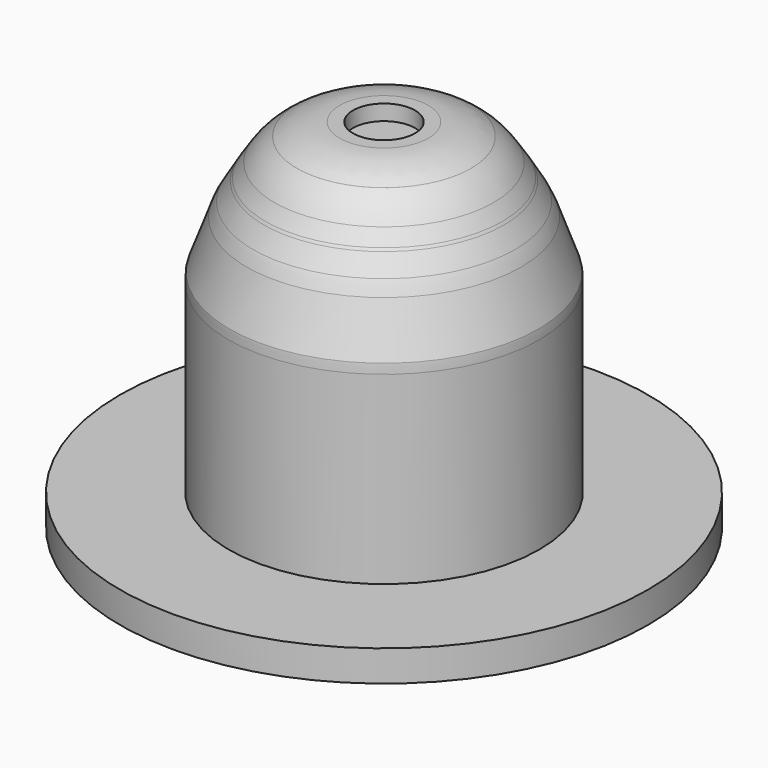
from build123d import *

# Parameters (mm, degrees)
F0_R     = 43.18
F0_R_2   = 25.4
F1_DEPTH = 5.08
F2_DEPTH = 36.83
F6_R     = 5.08
F7_DEPTH = 2.54


# Not quite as in the source:
# - a fillet or chamfer that OpenCascade refuses, or shapes differently, is made with other operations: its cross-section is extruded or revolved along the edge and cut away or added


with BuildPart() as f1:
    # F0 (on Top) → F1 (new body)
    with BuildSketch(Plane.XY):
        Circle(F0_R)
        Circle(F0_R_2, mode=Mode.SUBTRACT)
    extrude(amount=F1_DEPTH)

    # F0 (on Top) → F2 (join)
    with BuildSketch(Plane.XY):
        Circle(F0_R_2)
    extrude(amount=F2_DEPTH)

    # F3 (on Front) → F4 (revolve)
    with BuildSketch(Plane.XZ):
        Polygon((0, 58.42), (0, 36.8297025561), (25.3384895623, 36.7359854281), (22.0302641392, 45.9328517318), (19.5160117, 50.1673817635), (16.4724439383, 54.8650622368), (11.0508995131, 58.42), align=None)
    revolve(axis=Axis((0, 0, 47.6248512781), (0, 0, 1)))

    # F5: fillet of radius 12.7 on 5 edges, made by hand

    # F5_s1 → F5_t2 (revolve, cut)
    with BuildSketch(Plane.XZ):
        with BuildLine():
            ThreePointArc((25.4, 35.2768549118), (25.3761454392, 36.0548888463), (25.3046713696, 36.83))
            Line((25.3046713696, 36.83), (25.4, 36.83))
            Line((25.4, 36.83), (25.4, 35.2768549118))
        make_face()
    revolve(axis=Axis((0, 0, 36.83), (0, 0, 1)), mode=Mode.SUBTRACT)

    # F5_s3 → F5_t4 (revolve, cut)
    with BuildSketch(Plane.XZ):
        with BuildLine():
            ThreePointArc((19.6427134925, 49.9539892906), (19.513951513, 50.166103437), (19.3810699459, 50.3756614184))
            Line((19.3810699459, 50.3756614184), (19.5160117, 50.1673817635))
            Line((19.5160117, 50.1673817635), (19.6427134925, 49.9539892906))
        make_face()
    revolve(axis=Axis((0, 0, 50.1673817635), (0, 0, 1)), mode=Mode.SUBTRACT)

    # F5_s5 → F5_t6 (revolve, cut)
    with BuildSketch(Plane.XZ):
        with BuildLine():
            ThreePointArc((22.4409800917, 44.79106143), (21.9779508662, 45.9081881165), (21.4107694035, 46.9762111901))
            Line((21.4107694035, 46.9762111901), (22.0302641392, 45.9328517318))
            Line((22.0302641392, 45.9328517318), (22.4409800917, 44.79106143))
        make_face()
    revolve(axis=Axis((0, 0, 45.9328517318), (0, 0, 1)), mode=Mode.SUBTRACT)

    # F5_s7 → F5_t8 (revolve, cut)
    with BuildSketch(Plane.XZ):
        with BuildLine():
            ThreePointArc((17.9281816755, 52.6181627827), (16.274530798, 54.6682321185), (14.2335662066, 56.3331072017))
            Line((14.2335662066, 56.3331072017), (16.4724439383, 54.8650622368))
            Line((16.4724439383, 54.8650622368), (17.9281816755, 52.6181627827))
        make_face()
    revolve(axis=Axis((0, 0, 54.8650622368), (0, 0, 1)), mode=Mode.SUBTRACT)

    # F5_s9 → F5_t10 (revolve, cut)
    with BuildSketch(Plane.XZ):
        with BuildLine():
            ThreePointArc((14.2223539104, 56.3404591686), (10.8923380013, 57.8890145748), (7.2584579428, 58.42))
            Line((7.2584579428, 58.42), (11.0508995131, 58.42))
            Line((11.0508995131, 58.42), (14.2223539104, 56.3404591686))
        make_face()
    revolve(axis=Axis((0, 0, 58.42), (0, 0, 1)), mode=Mode.SUBTRACT)

    # F6 (on face) → F7 (cut)
    with BuildSketch(Plane.XY.offset(58.42)):
        Circle(F6_R)
    extrude(amount=-F7_DEPTH, mode=Mode.SUBTRACT)


solid = f1.part
